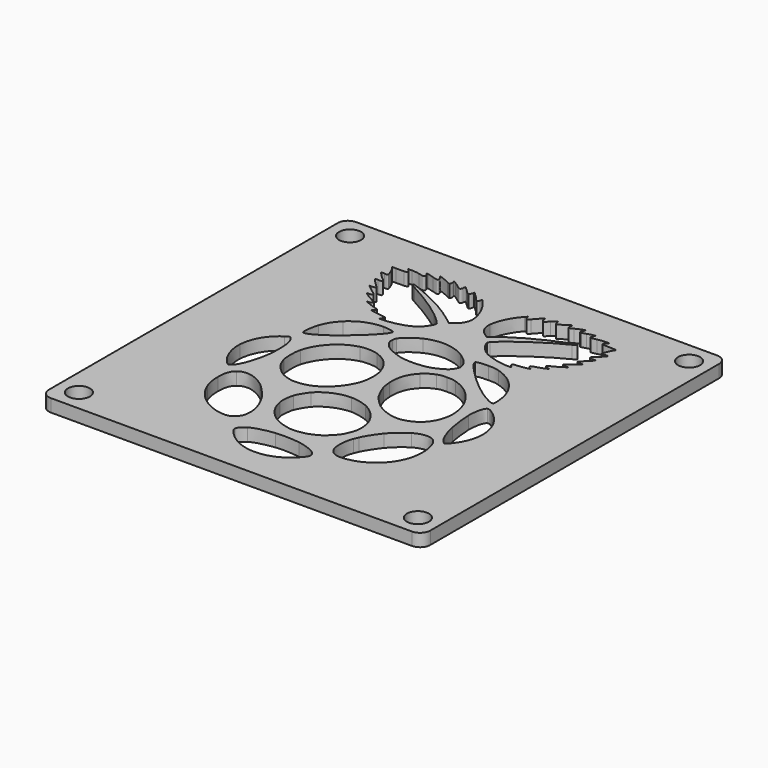
from build123d import *

# Parameters (mm, degrees)
F1_W     = 45
F1_H     = 45
F3_DEPTH = 1.5
F0_W     = 40
F0_H     = 40
F4_DEPTH = 1.5
F2_R     = 1.3
F5_DEPTH = 1.5
F6_R     = 1.2
F9_DEPTH = 28


# Not quite as in the source:
# - ends of sketch curves that miss each other by under 0.0002 mm in the source are joined
# - a feature names something its author has since deleted; it is built from what else it names


with BuildPart() as f3:
    # F1 (on Top) → F3 (new body)
    with BuildSketch(Plane.XY):
        Rectangle(F1_W, F1_H)
    extrude(amount=F3_DEPTH)

    # F0 (on Top) → F4 (join)
    with BuildSketch(Plane.XY):
        Rectangle(F0_W, F0_H)
    extrude(amount=F4_DEPTH)

    # F2 (on Top) → F5 (cut)
    with BuildSketch(Plane.XY):
        with Locations((-20, 20)):
            Circle(F2_R)
        with Locations((20, 20)):
            Circle(F2_R)
        with Locations((-20, -20)):
            Circle(F2_R)
        with Locations((20, -20)):
            Circle(F2_R)
    extrude(amount=F5_DEPTH, mode=Mode.SUBTRACT)

    # F6
    f6_edges = [f3.edges().sort_by_distance(p)[0] for p in [
        (22.5, 22.5, 0.75),
        (-22.5, 22.5, 0.75),
        (-22.5, -22.5, 0.75),
        (22.5, -22.5, 0.75),
    ]]
    fillet(f6_edges, radius=F6_R)

    # F8 (on offset) → F9 (cut)
    with BuildSketch(Plane.XY.offset(25)):
        with BuildLine():
            add(Edge.make_bspline(
                [(-0.887177, -19.067709), (-1.37051, -18.963367), (-1.920806, -18.777216), (-2.274089, -18.598552)],
                knots=[0, 0, 0, 0, 1, 1, 1, 1], degree=3))
            add(Edge.make_bspline(
                [(1.459681, -18.954491), (0.830557, -19.140329), (-0.298485, -19.194797), (-0.887177, -19.067709)],
                knots=[0, 0, 0, 0, 1, 1, 1, 1], degree=3))
            add(Edge.make_bspline(
                [(4.270525, -17.044889), (3.53259, -17.978447), (2.585341, -18.621978), (1.459681, -18.954491)],
                knots=[0, 0, 0, 0, 1, 1, 1, 1], degree=3))
            add(Edge.make_bspline(
                [(4.151263, -15.845306), (4.621657, -16.247946), (4.652807, -16.561266), (4.270525, -17.044889)],
                knots=[0, 0, 0, 0, 1, 1, 1, 1], degree=3))
            add(Edge.make_bspline(
                [(2.0744, -15.096764), (2.83072, -15.220852), (3.85158, -15.588789), (4.151263, -15.845306)],
                knots=[0, 0, 0, 0, 1, 1, 1, 1], degree=3))
            add(Edge.make_bspline(
                [(-0.779595, -15.005754), (-0.110166, -14.926798), (1.315549, -14.972262), (2.0744, -15.096764)],
                knots=[0, 0, 0, 0, 1, 1, 1, 1], degree=3))
            add(Edge.make_bspline(
                [(-3.491858, -15.740052), (-2.988685, -15.428195), (-1.929114, -15.141335), (-0.779595, -15.005754)],
                knots=[0, 0, 0, 0, 1, 1, 1, 1], degree=3))
            add(Edge.make_bspline(
                [(-4.28669, -16.671703), (-4.28669, -16.390931), (-4.000176, -16.055097), (-3.491858, -15.740052)],
                knots=[0, 0, 0, 0, 1, 1, 1, 1], degree=3))
            add(Edge.make_bspline(
                [(-2.274089, -18.598552), (-3.225122, -18.117593), (-4.28669, -17.101255), (-4.28669, -16.671703)],
                knots=[0, 0, 0, 0, 1, 1, 1, 1], degree=3))
        make_face()
        with BuildLine():
            add(Edge.make_bspline(
                [(-7.639187, -14.959263), (-9.375295, -14.593112), (-10.940378, -13.246308), (-11.591687, -11.558011)],
                knots=[0, 0, 0, 0, 1, 1, 1, 1], degree=3))
            add(Edge.make_bspline(
                [(-5.614103, -14.513096), (-6.04316, -15.058014), (-6.594745, -15.17954), (-7.639187, -14.959263)],
                knots=[0, 0, 0, 0, 1, 1, 1, 1], degree=3))
            add(Edge.make_bspline(
                [(-5.216704, -13.342755), (-5.262075, -13.965348), (-5.322169, -14.142328), (-5.614103, -14.513096)],
                knots=[0, 0, 0, 0, 1, 1, 1, 1], degree=3))
            add(Edge.make_bspline(
                [(-6.300441, -10.132584), (-5.552084, -11.291625), (-5.153311, -12.472844), (-5.216704, -13.342755)],
                knots=[0, 0, 0, 0, 1, 1, 1, 1], degree=3))
            add(Edge.make_bspline(
                [(-8.076125, -8.223123), (-7.617712, -8.559281), (-6.631616, -9.619669), (-6.300441, -10.132584)],
                knots=[0, 0, 0, 0, 1, 1, 1, 1], degree=3))
            add(Edge.make_bspline(
                [(-11.303389, -7.648184), (-10.556755, -7.048173), (-9.396515, -7.25487), (-8.076125, -8.223123)],
                knots=[0, 0, 0, 0, 1, 1, 1, 1], degree=3))
            add(Edge.make_bspline(
                [(-11.941857, -9.574962), (-11.939052, -8.581512), (-11.748239, -8.005675), (-11.303389, -7.648184)],
                knots=[0, 0, 0, 0, 1, 1, 1, 1], degree=3))
            add(Edge.make_bspline(
                [(-11.591687, -11.558011), (-11.837351, -10.921211), (-11.943954, -10.317508), (-11.941857, -9.574962)],
                knots=[0, 0, 0, 0, 1, 1, 1, 1], degree=3))
        make_face()
        with BuildLine():
            add(Edge.make_bspline(
                [(6.262145, -14.967016), (5.893137, -14.834758), (5.613918, -14.573111), (5.421003, -14.178806)],
                knots=[0, 0, 0, 0, 1, 1, 1, 1], degree=3))
            add(Edge.make_bspline(
                [(9.133644, -14.48583), (8.168538, -14.965389), (6.866406, -15.183591), (6.262145, -14.967016)],
                knots=[0, 0, 0, 0, 1, 1, 1, 1], degree=3))
            add(Edge.make_bspline(
                [(12.006219, -11.072921), (11.551716, -12.598138), (10.559015, -13.777568), (9.133644, -14.48583)],
                knots=[0, 0, 0, 0, 1, 1, 1, 1], degree=3))
            add(Edge.make_bspline(
                [(12.14776, -8.711004), (12.258855, -9.290003), (12.18871, -10.460516), (12.006219, -11.072921)],
                knots=[0, 0, 0, 0, 1, 1, 1, 1], degree=3))
            add(Edge.make_bspline(
                [(11.526211, -7.150542), (11.813997, -7.460815), (11.995142, -7.9156), (12.14776, -8.711004)],
                knots=[0, 0, 0, 0, 1, 1, 1, 1], degree=3))
            add(Edge.make_bspline(
                [(8.99643, -7.173879), (10.018251, -6.600622), (11.00768, -6.591495), (11.526211, -7.150542)],
                knots=[0, 0, 0, 0, 1, 1, 1, 1], degree=3))
            add(Edge.make_bspline(
                [(7.068817, -8.843622), (7.543457, -8.265319), (8.448742, -7.48114), (8.99643, -7.173879)],
                knots=[0, 0, 0, 0, 1, 1, 1, 1], degree=3))
            add(Edge.make_bspline(
                [(5.764471, -10.890116), (5.947246, -10.444129), (6.614661, -9.396967), (7.068817, -8.843622)],
                knots=[0, 0, 0, 0, 1, 1, 1, 1], degree=3))
            add(Edge.make_bspline(
                [(5.537969, -11.433611), (5.582241, -11.330639), (5.684167, -11.086066), (5.764471, -10.890116)],
                knots=[0, 0, 0, 0, 1, 1, 1, 1], degree=3))
            add(Edge.make_bspline(
                [(5.421003, -14.178806), (5.139993, -13.604443), (5.198884, -12.222282), (5.537969, -11.433611)],
                knots=[0, 0, 0, 0, 1, 1, 1, 1], degree=3))
        make_face()
        with BuildLine():
            add(Edge.make_bspline(
                [(-0.235604, -13.50576), (-1.520983, -13.321682), (-2.446325, -12.892636), (-3.164632, -12.147682)],
                knots=[0, 0, 0, 0, 1, 1, 1, 1], degree=3))
            add(Edge.make_bspline(
                [(1.294176, -13.368537), (0.827588, -13.48029), (0.064506, -13.548739), (-0.235604, -13.50576)],
                knots=[0, 0, 0, 0, 1, 1, 1, 1], degree=3))
            add(Edge.make_bspline(
                [(2.342359, -12.964243), (2.015156, -13.126896), (1.543474, -13.308828), (1.294176, -13.368537)],
                knots=[0, 0, 0, 0, 1, 1, 1, 1], degree=3))
            add(Edge.make_bspline(
                [(3.504831, -12.099096), (3.002423, -12.603148), (2.868984, -12.702458), (2.342359, -12.964243)],
                knots=[0, 0, 0, 0, 1, 1, 1, 1], degree=3))
            add(Edge.make_bspline(
                [(4.310692, -11.042532), (4.112024, -11.448654), (3.977986, -11.624393), (3.504831, -12.099096)],
                knots=[0, 0, 0, 0, 1, 1, 1, 1], degree=3))
            add(Edge.make_bspline(
                [(4.7003, -8.628597), (4.848256, -9.47946), (4.736451, -10.172181), (4.310692, -11.042532)],
                knots=[0, 0, 0, 0, 1, 1, 1, 1], degree=3))
            add(Edge.make_bspline(
                [(4.072547, -7.091122), (4.444928, -7.656361), (4.595264, -8.02456), (4.7003, -8.628597)],
                knots=[0, 0, 0, 0, 1, 1, 1, 1], degree=3))
            add(Edge.make_bspline(
                [(2.200713, -5.511063), (2.857354, -5.7868), (3.659134, -6.463601), (4.072547, -7.091122)],
                knots=[0, 0, 0, 0, 1, 1, 1, 1], degree=3))
            add(Edge.make_bspline(
                [(0.257769, -5.098998), (0.762084, -5.099054), (1.686404, -5.295094), (2.200713, -5.511063)],
                knots=[0, 0, 0, 0, 1, 1, 1, 1], degree=3))
            add(Edge.make_bspline(
                [(-3.303441, -6.648636), (-2.500624, -5.733191), (-1.042809, -5.098832), (0.257769, -5.098998)],
                knots=[0, 0, 0, 0, 1, 1, 1, 1], degree=3))
            add(Edge.make_bspline(
                [(-4.1749, -8.134608), (-4.037742, -7.735953), (-3.595159, -6.98128), (-3.303441, -6.648636)],
                knots=[0, 0, 0, 0, 1, 1, 1, 1], degree=3))
            add(Edge.make_bspline(
                [(-4.339107, -9.886584), (-4.409434, -9.514024), (-4.319552, -8.555046), (-4.1749, -8.134608)],
                knots=[0, 0, 0, 0, 1, 1, 1, 1], degree=3))
            add(Edge.make_bspline(
                [(-3.164632, -12.147682), (-3.832592, -11.454942), (-4.163202, -10.818452), (-4.339107, -9.886584)],
                knots=[0, 0, 0, 0, 1, 1, 1, 1], degree=3))
        make_face()
        with BuildLine():
            add(Edge.make_bspline(
                [(-13.180571, -6.694966), (-13.990038, -5.840955), (-14.48352, -4.449729), (-14.40991, -3.229206)],
                knots=[0, 0, 0, 0, 1, 1, 1, 1], degree=3))
            add(Edge.make_bspline(
                [(-12.795313, -7.025328), (-12.834983, -7.025328), (-13.008349, -6.876665), (-13.180571, -6.694966)],
                knots=[0, 0, 0, 0, 1, 1, 1, 1], degree=3))
            add(Edge.make_bspline(
                [(-11.056067, -2.860925), (-11.378643, -5.18677), (-12.146509, -7.025328), (-12.795313, -7.025328)],
                knots=[0, 0, 0, 0, 1, 1, 1, 1], degree=3))
            add(Edge.make_bspline(
                [(-11.089866, -0.450994), (-11.017705, -0.916083), (-10.996457, -2.431121), (-11.056067, -2.860925)],
                knots=[0, 0, 0, 0, 1, 1, 1, 1], degree=3))
            add(Edge.make_bspline(
                [(-11.767433, 0.793551), (-11.50836, 0.793551), (-11.193126, 0.214534), (-11.089866, -0.450994)],
                knots=[0, 0, 0, 0, 1, 1, 1, 1], degree=3))
            add(Edge.make_bspline(
                [(-12.195937, 0.576602), (-12.011923, 0.695924), (-11.819096, 0.793551), (-11.767433, 0.793551)],
                knots=[0, 0, 0, 0, 1, 1, 1, 1], degree=3))
            add(Edge.make_bspline(
                [(-14.40991, -3.229206), (-14.317171, -1.691471), (-13.483414, -0.258248), (-12.195937, 0.576602)],
                knots=[0, 0, 0, 0, 1, 1, 1, 1], degree=3))
        make_face()
        with BuildLine():
            add(Edge.make_bspline(
                [(12.400777, -6.735775), (11.971045, -6.358465), (11.479362, -5.183704), (11.231968, -3.943179)],
                knots=[0, 0, 0, 0, 1, 1, 1, 1], degree=3))
            add(Edge.make_bspline(
                [(12.643578, -6.912011), (12.620435, -6.912011), (12.511174, -6.832705), (12.400777, -6.735775)],
                knots=[0, 0, 0, 0, 1, 1, 1, 1], degree=3))
            add(Edge.make_bspline(
                [(13.724147, -5.604577), (13.393346, -6.220246), (12.821615, -6.912011), (12.643578, -6.912011)],
                knots=[0, 0, 0, 0, 1, 1, 1, 1], degree=3))
            add(Edge.make_bspline(
                [(12.291561, 0.591731), (14.29644, -0.911772), (14.882837, -3.448092), (13.724147, -5.604577)],
                knots=[0, 0, 0, 0, 1, 1, 1, 1], degree=3))
            add(Edge.make_bspline(
                [(11.424514, 0.968577), (11.585105, 1.041747), (11.838113, 0.931782), (12.291561, 0.591731)],
                knots=[0, 0, 0, 0, 1, 1, 1, 1], degree=3))
            add(Edge.make_bspline(
                [(10.897877, -1.140843), (10.89799, -0.089468), (11.128489, 0.833699), (11.424514, 0.968577)],
                knots=[0, 0, 0, 0, 1, 1, 1, 1], degree=3))
            add(Edge.make_bspline(
                [(11.231968, -3.943179), (11.042484, -2.99304), (10.897795, -1.779392), (10.897877, -1.140843)],
                knots=[0, 0, 0, 0, 1, 1, 1, 1], degree=3))
        make_face()
        with BuildLine():
            add(Edge.make_bspline(
                [(-6.666349, -5.76274), (-7.397165, -5.563072), (-7.812664, -5.318386), (-8.366105, -4.761759)],
                knots=[0, 0, 0, 0, 1, 1, 1, 1], degree=3))
            add(Edge.make_bspline(
                [(-5.589836, -5.868818), (-6.089609, -5.890241), (-6.261771, -5.873277), (-6.666349, -5.76274)],
                knots=[0, 0, 0, 0, 1, 1, 1, 1], degree=3))
            add(Edge.make_bspline(
                [(-3.037567, -4.927008), (-3.859885, -5.536619), (-4.651088, -5.828579), (-5.589836, -5.868818)],
                knots=[0, 0, 0, 0, 1, 1, 1, 1], degree=3))
            add(Edge.make_bspline(
                [(-1.048832, -2.213387), (-1.399312, -3.231715), (-2.170865, -4.284496), (-3.037567, -4.927008)],
                knots=[0, 0, 0, 0, 1, 1, 1, 1], degree=3))
            add(Edge.make_bspline(
                [(-0.96737, 0.699644), (-0.703326, -0.086928), (-0.737495, -1.308792), (-1.048832, -2.213387)],
                knots=[0, 0, 0, 0, 1, 1, 1, 1], degree=3))
            add(Edge.make_bspline(
                [(-3.42309, 3.239768), (-2.143037, 2.780187), (-1.411922, 2.023944), (-0.96737, 0.699644)],
                knots=[0, 0, 0, 0, 1, 1, 1, 1], degree=3))
            add(Edge.make_bspline(
                [(-5.480047, 3.292589), (-4.869522, 3.44673), (-3.932516, 3.422668), (-3.42309, 3.239768)],
                knots=[0, 0, 0, 0, 1, 1, 1, 1], degree=3))
            add(Edge.make_bspline(
                [(-9.344396, -0.617591), (-8.788871, 1.322296), (-7.294369, 2.834522), (-5.480047, 3.292589)],
                knots=[0, 0, 0, 0, 1, 1, 1, 1], degree=3))
            add(Edge.make_bspline(
                [(-9.366706, -3.05923), (-9.521893, -2.499388), (-9.509981, -1.195815), (-9.344396, -0.617591)],
                knots=[0, 0, 0, 0, 1, 1, 1, 1], degree=3))
            add(Edge.make_bspline(
                [(-8.366105, -4.761759), (-8.890736, -4.234108), (-9.175204, -3.750084), (-9.366706, -3.05923)],
                knots=[0, 0, 0, 0, 1, 1, 1, 1], degree=3))
        make_face()
        with BuildLine():
            add(Edge.make_bspline(
                [(5.685213, -5.683681), (4.999679, -5.613281), (4.164647, -5.284724), (3.47553, -4.814245)],
                knots=[0, 0, 0, 0, 1, 1, 1, 1], degree=3))
            add(Edge.make_bspline(
                [(6.77887, -5.631059), (6.39194, -5.717519), (6.135065, -5.729879), (5.685213, -5.683681)],
                knots=[0, 0, 0, 0, 1, 1, 1, 1], degree=3))
            add(Edge.make_bspline(
                [(9.388712, -0.341026), (10.142836, -2.830944), (9.00703, -5.133173), (6.77887, -5.631059)],
                knots=[0, 0, 0, 0, 1, 1, 1, 1], degree=3))
            add(Edge.make_bspline(
                [(5.739077, 3.408924), (7.469211, 2.86561), (8.84595, 1.451029), (9.388712, -0.341026)],
                knots=[0, 0, 0, 0, 1, 1, 1, 1], degree=3))
            add(Edge.make_bspline(
                [(4.608701, 3.538068), (5.19957, 3.540923), (5.386887, 3.519522), (5.739077, 3.408924)],
                knots=[0, 0, 0, 0, 1, 1, 1, 1], degree=3))
            add(Edge.make_bspline(
                [(3.509753, 3.381682), (3.857557, 3.517846), (3.978255, 3.535021), (4.608701, 3.538068)],
                knots=[0, 0, 0, 0, 1, 1, 1, 1], degree=3))
            add(Edge.make_bspline(
                [(2.221864, 2.567223), (2.575367, 2.931901), (2.92395, 3.152344), (3.509753, 3.381682)],
                knots=[0, 0, 0, 0, 1, 1, 1, 1], degree=3))
            add(Edge.make_bspline(
                [(1.115416, -0.566001), (1.045522, 0.71934), (1.397906, 1.717218), (2.221864, 2.567223)],
                knots=[0, 0, 0, 0, 1, 1, 1, 1], degree=3))
            add(Edge.make_bspline(
                [(1.256315, -1.614437), (1.198315, -1.396302), (1.13491, -0.924506), (1.115416, -0.566001)],
                knots=[0, 0, 0, 0, 1, 1, 1, 1], degree=3))
            add(Edge.make_bspline(
                [(2.15982, -3.512498), (1.91394, -3.182298), (1.368556, -2.036567), (1.256315, -1.614437)],
                knots=[0, 0, 0, 0, 1, 1, 1, 1], degree=3))
            add(Edge.make_bspline(
                [(3.47553, -4.814245), (3.1611, -4.599576), (2.432554, -3.878762), (2.15982, -3.512498)],
                knots=[0, 0, 0, 0, 1, 1, 1, 1], degree=3))
        make_face()
        with BuildLine():
            add(Edge.make_bspline(
                [(10.416201, 2.345395), (9.765312, 2.693907), (9.335171, 2.964027), (8.91475, 3.288278)],
                knots=[0, 0, 0, 0, 1, 1, 1, 1], degree=3))
            add(Edge.make_bspline(
                [(11.216192, 2.245104), (11.162124, 2.029681), (10.958074, 2.055262), (10.416201, 2.345395)],
                knots=[0, 0, 0, 0, 1, 1, 1, 1], degree=3))
            add(Edge.make_bspline(
                [(11.216588, 2.882513), (11.236851, 2.613562), (11.236667, 2.326728), (11.216192, 2.245104)],
                knots=[0, 0, 0, 0, 1, 1, 1, 1], degree=3))
            add(Edge.make_bspline(
                [(7.458432, 7.572423), (9.62561, 6.916458), (11.046244, 5.143608), (11.216588, 2.882513)],
                knots=[0, 0, 0, 0, 1, 1, 1, 1], degree=3))
            add(Edge.make_bspline(
                [(6.166811, 7.728751), (6.853439, 7.724014), (7.027005, 7.703009), (7.458432, 7.572423)],
                knots=[0, 0, 0, 0, 1, 1, 1, 1], degree=3))
            add(Edge.make_bspline(
                [(4.741901, 7.506008), (4.796308, 7.647789), (5.350255, 7.734383), (6.166811, 7.728751)],
                knots=[0, 0, 0, 0, 1, 1, 1, 1], degree=3))
            add(Edge.make_bspline(
                [(5.110777, 6.799356), (4.858896, 7.113128), (4.70458, 7.40875), (4.741901, 7.506008)],
                knots=[0, 0, 0, 0, 1, 1, 1, 1], degree=3))
            add(Edge.make_bspline(
                [(8.036543, 3.958679), (7.279806, 4.532045), (5.697985, 6.067863), (5.110777, 6.799356)],
                knots=[0, 0, 0, 0, 1, 1, 1, 1], degree=3))
            add(Edge.make_bspline(
                [(8.91475, 3.288278), (8.712196, 3.444499), (8.317003, 3.746179), (8.036543, 3.958679)],
                knots=[0, 0, 0, 0, 1, 1, 1, 1], degree=3))
        make_face()
        with BuildLine():
            add(Edge.make_bspline(
                [(-11.391275, 2.299636), (-11.494252, 2.56799), (-11.354362, 3.602861), (-11.123694, 4.279138)],
                knots=[0, 0, 0, 0, 1, 1, 1, 1], degree=3))
            add(Edge.make_bspline(
                [(-11.232042, 2.210014), (-11.300705, 2.210014), (-11.37236, 2.250344), (-11.391275, 2.299636)],
                knots=[0, 0, 0, 0, 1, 1, 1, 1], degree=3))
            add(Edge.make_bspline(
                [(-10.112701, 2.674987), (-10.455355, 2.455288), (-11.04581, 2.210014), (-11.232042, 2.210014)],
                knots=[0, 0, 0, 0, 1, 1, 1, 1], degree=3))
            add(Edge.make_bspline(
                [(-9.499276, 3.055627), (-9.670668, 2.952703), (-9.946709, 2.781416), (-10.112701, 2.674987)],
                knots=[0, 0, 0, 0, 1, 1, 1, 1], degree=3))
            add(Edge.make_bspline(
                [(-6.639739, 5.362827), (-7.53775, 4.527583), (-8.962803, 3.377787), (-9.499276, 3.055627)],
                knots=[0, 0, 0, 0, 1, 1, 1, 1], degree=3))
            add(Edge.make_bspline(
                [(-4.957272, 7.54926), (-4.778051, 7.370039), (-5.524177, 6.400419), (-6.639739, 5.362827)],
                knots=[0, 0, 0, 0, 1, 1, 1, 1], degree=3))
            add(Edge.make_bspline(
                [(-6.25059, 7.760561), (-5.723939, 7.758544), (-5.057705, 7.649693), (-4.957272, 7.54926)],
                knots=[0, 0, 0, 0, 1, 1, 1, 1], degree=3))
            add(Edge.make_bspline(
                [(-9.844138, 6.291024), (-8.887425, 7.240353), (-7.602654, 7.765745), (-6.25059, 7.760561)],
                knots=[0, 0, 0, 0, 1, 1, 1, 1], degree=3))
            add(Edge.make_bspline(
                [(-11.123694, 4.279138), (-10.854269, 5.069039), (-10.475596, 5.664438), (-9.844138, 6.291024)],
                knots=[0, 0, 0, 0, 1, 1, 1, 1], degree=3))
        make_face()
        with BuildLine():
            add(Edge.make_bspline(
                [(-0.75693, 3.913219), (-1.661555, 4.030979), (-2.894979, 4.537561), (-3.41168, 5.003555)],
                knots=[0, 0, 0, 0, 1, 1, 1, 1], degree=3))
            add(Edge.make_bspline(
                [(1.605798, 3.971855), (0.922233, 3.846833), (-0.059754, 3.822463), (-0.75693, 3.913219)],
                knots=[0, 0, 0, 0, 1, 1, 1, 1], degree=3))
            add(Edge.make_bspline(
                [(2.943425, 4.422067), (2.374586, 4.147585), (2.146049, 4.070665), (1.605798, 3.971855)],
                knots=[0, 0, 0, 0, 1, 1, 1, 1], degree=3))
            add(Edge.make_bspline(
                [(4.216517, 5.578006), (3.980659, 5.04481), (3.693325, 4.783917), (2.943425, 4.422067)],
                knots=[0, 0, 0, 0, 1, 1, 1, 1], degree=3))
            add(Edge.make_bspline(
                [(4.268538, 6.148803), (4.325273, 5.875514), (4.319344, 5.810464), (4.216517, 5.578006)],
                knots=[0, 0, 0, 0, 1, 1, 1, 1], degree=3))
            add(Edge.make_bspline(
                [(2.771734, 7.847433), (3.594347, 7.321914), (4.157729, 6.682567), (4.268538, 6.148803)],
                knots=[0, 0, 0, 0, 1, 1, 1, 1], degree=3))
            add(Edge.make_bspline(
                [(-1.943801, 8.212033), (-0.42835, 8.89197), (1.352178, 8.754301), (2.771734, 7.847433)],
                knots=[0, 0, 0, 0, 1, 1, 1, 1], degree=3))
            add(Edge.make_bspline(
                [(-3.858635, 6.692064), (-3.620796, 7.151995), (-2.729441, 7.85954), (-1.943801, 8.212033)],
                knots=[0, 0, 0, 0, 1, 1, 1, 1], degree=3))
            add(Edge.make_bspline(
                [(-3.987133, 6.204006), (-3.970143, 6.368625), (-3.912319, 6.588251), (-3.858635, 6.692064)],
                knots=[0, 0, 0, 0, 1, 1, 1, 1], degree=3))
            add(Edge.make_bspline(
                [(-3.8549, 5.580431), (-3.993254, 5.85546), (-4.013333, 5.950149), (-3.987133, 6.204006)],
                knots=[0, 0, 0, 0, 1, 1, 1, 1], degree=3))
            add(Edge.make_bspline(
                [(-3.41168, 5.003555), (-3.567636, 5.144205), (-3.764073, 5.399879), (-3.8549, 5.580431)],
                knots=[0, 0, 0, 0, 1, 1, 1, 1], degree=3))
        make_face()
        with BuildLine():
            add(Edge.make_bspline(
                [(-7.583908, 8.810406), (-7.605552, 8.833099), (-7.548185, 8.914838), (-7.456426, 8.992048)],
                knots=[0, 0, 0, 0, 1, 1, 1, 1], degree=3))
            add(Edge.make_bspline(
                [(-5.9005, 8.955461), (-6.468685, 8.832359), (-7.518565, 8.741893), (-7.583908, 8.810406)],
                knots=[0, 0, 0, 0, 1, 1, 1, 1], degree=3))
            add(Edge.make_bspline(
                [(-3.247876, 10.382302), (-3.752675, 9.672456), (-4.536049, 9.25108), (-5.9005, 8.955461)],
                knots=[0, 0, 0, 0, 1, 1, 1, 1], degree=3))
            add(Edge.make_bspline(
                [(-2.813568, 11.274492), (-2.813568, 11.104658), (-2.985819, 10.750807), (-3.247876, 10.382302)],
                knots=[0, 0, 0, 0, 1, 1, 1, 1], degree=3))
            add(Edge.make_bspline(
                [(-4.173373, 12.612296), (-3.530382, 12.090563), (-2.813568, 11.385346), (-2.813568, 11.274492)],
                knots=[0, 0, 0, 0, 1, 1, 1, 1], degree=3))
            add(Edge.make_bspline(
                [(-8.975184, 15.695384), (-7.157498, 14.731691), (-5.374354, 13.586791), (-4.173373, 12.612296)],
                knots=[0, 0, 0, 0, 1, 1, 1, 1], degree=3))
            add(Edge.make_bspline(
                [(-9.326446, 16.091357), (-9.566099, 16.091357), (-9.427627, 15.935259), (-8.975184, 15.695384)],
                knots=[0, 0, 0, 0, 1, 1, 1, 1], degree=3))
            add(Edge.make_bspline(
                [(-5.191011, 14.250973), (-6.397057, 14.923274), (-9.021798, 16.091357), (-9.326446, 16.091357)],
                knots=[0, 0, 0, 0, 1, 1, 1, 1], degree=3))
            add(Edge.make_bspline(
                [(-2.542429, 12.503854), (-3.10486, 12.95853), (-4.372307, 13.794593), (-5.191011, 14.250973)],
                knots=[0, 0, 0, 0, 1, 1, 1, 1], degree=3))
            Line((-2.542429, 12.503854), (-1.777539, 12.316211))
            add(Edge.make_bspline(
                [(-0.754494, 14.020254), (-0.756041, 13.332166), (-1.102995, 12.754256), (-1.777539, 12.316211)],
                knots=[0, 0, 0, 0, 1, 1, 1, 1], degree=3))
            add(Edge.make_bspline(
                [(-2.236226, 17.343044), (-1.406614, 16.440804), (-0.752353, 14.973619), (-0.754494, 14.020254)],
                knots=[0, 0, 0, 0, 1, 1, 1, 1], degree=3))
            Line((-2.236226, 17.343044), (-2.597227, 17.391871))
            add(Edge.make_bspline(
                [(-2.762855, 17.123708), (-2.718006, 17.132415), (-2.643474, 17.253089), (-2.597227, 17.391871)],
                knots=[0, 0, 0, 0, 1, 1, 1, 1], degree=3))
            add(Edge.make_bspline(
                [(-3.052306, 17.378671), (-2.937957, 17.229733), (-2.807704, 17.115), (-2.762855, 17.123708)],
                knots=[0, 0, 0, 0, 1, 1, 1, 1], degree=3))
            add(Edge.make_bspline(
                [(-4.023399, 18.314751), (-4.060666, 18.457259), (-3.36715, 17.788748), (-3.052306, 17.378671)],
                knots=[0, 0, 0, 0, 1, 1, 1, 1], degree=3))
            add(Edge.make_bspline(
                [(-4.22542, 17.764247), (-4.104771, 17.80254), (-3.979045, 18.14514), (-4.023399, 18.314751)],
                knots=[0, 0, 0, 0, 1, 1, 1, 1], degree=3))
            add(Edge.make_bspline(
                [(-4.781638, 18.186479), (-4.451461, 17.856302), (-4.299304, 17.740797), (-4.22542, 17.764247)],
                knots=[0, 0, 0, 0, 1, 1, 1, 1], degree=3))
            add(Edge.make_bspline(
                [(-5.299676, 18.640991), (-5.264736, 18.640991), (-5.031619, 18.436461), (-4.781638, 18.186479)],
                knots=[0, 0, 0, 0, 1, 1, 1, 1], degree=3))
            add(Edge.make_bspline(
                [(-5.363202, 18.425689), (-5.363202, 18.546968), (-5.33546, 18.640991), (-5.299676, 18.640991)],
                knots=[0, 0, 0, 0, 1, 1, 1, 1], degree=3))
            add(Edge.make_bspline(
                [(-5.572553, 18.074406), (-5.441507, 18.074406), (-5.363202, 18.205798), (-5.363202, 18.425689)],
                knots=[0, 0, 0, 0, 1, 1, 1, 1], degree=3))
            add(Edge.make_bspline(
                [(-5.986628, 18.348948), (-5.799241, 18.19795), (-5.612907, 18.074406), (-5.572553, 18.074406)],
                knots=[0, 0, 0, 0, 1, 1, 1, 1], degree=3))
            add(Edge.make_bspline(
                [(-6.61564, 18.780407), (-6.457071, 18.694103), (-6.174015, 18.499946), (-5.986628, 18.348948)],
                knots=[0, 0, 0, 0, 1, 1, 1, 1], degree=3))
            add(Edge.make_bspline(
                [(-6.83853, 18.815089), (-6.900272, 18.930456), (-6.887747, 18.928507), (-6.61564, 18.780407)],
                knots=[0, 0, 0, 0, 1, 1, 1, 1], degree=3))
            add(Edge.make_bspline(
                [(-6.902968, 18.255668), (-6.785133, 18.277983), (-6.74368, 18.63786), (-6.83853, 18.815089)],
                knots=[0, 0, 0, 0, 1, 1, 1, 1], degree=3))
            add(Edge.make_bspline(
                [(-7.240947, 18.391086), (-7.107293, 18.306714), (-6.955202, 18.245776), (-6.902968, 18.255668)],
                knots=[0, 0, 0, 0, 1, 1, 1, 1], degree=3))
            add(Edge.make_bspline(
                [(-8.429431, 18.867625), (-8.298125, 18.867625), (-7.46955, 18.535397), (-7.240947, 18.391086)],
                knots=[0, 0, 0, 0, 1, 1, 1, 1], degree=3))
            add(Edge.make_bspline(
                [(-8.342812, 18.693302), (-8.423488, 18.78918), (-8.462466, 18.867625), (-8.429431, 18.867625)],
                knots=[0, 0, 0, 0, 1, 1, 1, 1], degree=3))
            add(Edge.make_bspline(
                [(-8.289421, 18.187723), (-8.140904, 18.187723), (-8.17298, 18.491468), (-8.342812, 18.693302)],
                knots=[0, 0, 0, 0, 1, 1, 1, 1], degree=3))
            add(Edge.make_bspline(
                [(-8.898501, 18.350774), (-8.614818, 18.261096), (-8.340733, 18.187723), (-8.289421, 18.187723)],
                knots=[0, 0, 0, 0, 1, 1, 1, 1], degree=3))
            add(Edge.make_bspline(
                [(-9.640922, 18.554087), (-9.516273, 18.531943), (-9.182184, 18.440451), (-8.898501, 18.350774)],
                knots=[0, 0, 0, 0, 1, 1, 1, 1], degree=3))
            Line((-9.640922, 18.554087), (-9.740074, 18.458208))
            add(Edge.make_bspline(
                [(-9.612593, 18.141577), (-9.612593, 18.25064), (-9.663042, 18.375942), (-9.740074, 18.458208)],
                knots=[0, 0, 0, 0, 1, 1, 1, 1], degree=3))
            add(Edge.make_bspline(
                [(-10.320824, 18.074406), (-9.68754, 17.912439), (-9.612593, 17.919547), (-9.612593, 18.141577)],
                knots=[0, 0, 0, 0, 1, 1, 1, 1], degree=3))
            add(Edge.make_bspline(
                [(-11.240458, 18.187723), (-10.949351, 18.187723), (-10.591467, 18.143624), (-10.320824, 18.074406)],
                knots=[0, 0, 0, 0, 1, 1, 1, 1], degree=3))
            Line((-11.240458, 18.187723), (-11.514688, 17.996892))
            add(Edge.make_bspline(
                [(-11.723123, 17.592696), (-11.239516, 17.637563), (-11.204888, 17.704713), (-11.514688, 17.996892)],
                knots=[0, 0, 0, 0, 1, 1, 1, 1], degree=3))
            add(Edge.make_bspline(
                [(-12.621958, 17.573698), (-12.353525, 17.563188), (-11.949049, 17.571738), (-11.723123, 17.592696)],
                knots=[0, 0, 0, 0, 1, 1, 1, 1], degree=3))
            Line((-12.621958, 17.573698), (-12.971257, 17.411168))
            add(Edge.make_bspline(
                [(-12.446212, 16.212238), (-12.447118, 16.387367), (-12.793659, 17.178693), (-12.971257, 17.411168)],
                knots=[0, 0, 0, 0, 1, 1, 1, 1], degree=3))
            add(Edge.make_bspline(
                [(-12.8138, 16.117595), (-12.453047, 16.078962), (-12.445534, 16.080896), (-12.446212, 16.212238)],
                knots=[0, 0, 0, 0, 1, 1, 1, 1], degree=3))
            add(Edge.make_bspline(
                [(-13.182081, 16.09166), (-13.182081, 16.138394), (-13.077069, 16.145789), (-12.8138, 16.117595)],
                knots=[0, 0, 0, 0, 1, 1, 1, 1], degree=3))
            add(Edge.make_bspline(
                [(-12.336475, 15.213148), (-12.624692, 15.424566), (-13.182081, 16.003644), (-13.182081, 16.09166)],
                knots=[0, 0, 0, 0, 1, 1, 1, 1], degree=3))
            add(Edge.make_bspline(
                [(-12.119325, 14.901526), (-12.108141, 15.010242), (-12.158624, 15.082688), (-12.336475, 15.213148)],
                knots=[0, 0, 0, 0, 1, 1, 1, 1], degree=3))
            add(Edge.make_bspline(
                [(-12.510271, 14.759879), (-12.150465, 14.759879), (-12.133256, 14.766114), (-12.119325, 14.901526)],
                knots=[0, 0, 0, 0, 1, 1, 1, 1], degree=3))
            Line((-12.510271, 14.759879), (-12.776285, 14.605113))
            add(Edge.make_bspline(
                [(-12.187888, 14.010198), (-12.450809, 14.25228), (-12.715587, 14.519992), (-12.776285, 14.605113)],
                knots=[0, 0, 0, 0, 1, 1, 1, 1], degree=3))
            add(Edge.make_bspline(
                [(-11.709405, 13.505289), (-11.709631, 13.540907), (-11.924968, 13.768117), (-12.187888, 14.010198)],
                knots=[0, 0, 0, 0, 1, 1, 1, 1], degree=3))
            add(Edge.make_bspline(
                [(-12.152697, 13.369329), (-11.845722, 13.372134), (-11.708777, 13.414135), (-11.709405, 13.505289)],
                knots=[0, 0, 0, 0, 1, 1, 1, 1], degree=3))
            Line((-12.152697, 13.369329), (-12.162227, 13.140631))
            add(Edge.make_bspline(
                [(-11.470076, 12.618957), (-11.710529, 12.78142), (-12.021997, 13.016174), (-12.162227, 13.140631)],
                knots=[0, 0, 0, 0, 1, 1, 1, 1], degree=3))
            add(Edge.make_bspline(
                [(-11.444465, 12.066565), (-10.888261, 12.071364), (-10.895655, 12.230844), (-11.470076, 12.618957)],
                knots=[0, 0, 0, 0, 1, 1, 1, 1], degree=3))
            Line((-11.444465, 12.066565), (-11.510654, 11.923649))
            add(Edge.make_bspline(
                [(-10.240111, 11.17892), (-10.52654, 11.291433), (-11.28244, 11.734503), (-11.510654, 11.923649)],
                knots=[0, 0, 0, 0, 1, 1, 1, 1], degree=3))
            add(Edge.make_bspline(
                [(-10.480324, 10.76295), (-9.991013, 10.769741), (-9.844469, 11.023507), (-10.240111, 11.17892)],
                knots=[0, 0, 0, 0, 1, 1, 1, 1], degree=3))
            Line((-10.480324, 10.76295), (-10.462471, 10.655618))
            add(Edge.make_bspline(
                [(-8.989349, 10.145724), (-9.54331, 10.307189), (-10.296553, 10.567911), (-10.462471, 10.655618)],
                knots=[0, 0, 0, 0, 1, 1, 1, 1], degree=3))
            add(Edge.make_bspline(
                [(-9.074337, 9.776533), (-8.808668, 9.906316), (-8.768382, 10.081318), (-8.989349, 10.145724)],
                knots=[0, 0, 0, 0, 1, 1, 1, 1], degree=3))
            Line((-9.074337, 9.776533), (-9.046007, 9.590982))
            add(Edge.make_bspline(
                [(-8.224458, 9.456601), (-8.53608, 9.489351), (-8.905777, 9.549822), (-9.046007, 9.590982)],
                knots=[0, 0, 0, 0, 1, 1, 1, 1], degree=3))
            add(Edge.make_bspline(
                [(-7.289593, 9.238142), (-7.289593, 9.355611), (-7.310923, 9.360596), (-8.224458, 9.456601)],
                knots=[0, 0, 0, 0, 1, 1, 1, 1], degree=3))
            add(Edge.make_bspline(
                [(-7.456426, 8.992048), (-7.364668, 9.069258), (-7.289593, 9.18), (-7.289593, 9.238142)],
                knots=[0, 0, 0, 0, 1, 1, 1, 1], degree=3))
        make_face()
        Polygon((-9.300971, 9.66582), (-9.046007, 9.590982), (-9.074337, 9.776533), align=None)
        Polygon((-10.660776, 10.760446), (-10.462471, 10.655618), (-10.480324, 10.76295), align=None)
        Polygon((-1.777539, 12.316211), (-2.542429, 12.503854), (-2.072986, 12.124349), align=None)
        Polygon((-11.680629, 12.064525), (-11.510654, 11.923649), (-11.444465, 12.066565), align=None)
        Polygon((-2.597227, 17.391871), (-2.236226, 17.343044), (-2.513143, 17.644203), align=None)
        Polygon((-12.41719, 13.366915), (-12.162227, 13.140631), (-12.152697, 13.369329), align=None)
        Polygon((-12.886644, 14.759879), (-12.776285, 14.605113), (-12.510271, 14.759879), align=None)
        Polygon((-13.11002, 17.592808), (-12.971257, 17.411168), (-12.621958, 17.573698), align=None)
        Polygon((-11.717027, 18.187723), (-11.514688, 17.996892), (-11.240458, 18.187723), align=None)
        Polygon((-9.740074, 18.458208), (-9.640922, 18.554087), (-9.867556, 18.59435), align=None)
        with BuildLine():
            add(Edge.make_bspline(
                [(6.678906, 8.872284), (6.000035, 8.977778), (5.237201, 9.200614), (4.738118, 9.439219)],
                knots=[0, 0, 0, 0, 1, 1, 1, 1], degree=3))
            add(Edge.make_bspline(
                [(7.970238, 8.819974), (7.90965, 8.759386), (7.227638, 8.787013), (6.678906, 8.872284)],
                knots=[0, 0, 0, 0, 1, 1, 1, 1], degree=3))
            add(Edge.make_bspline(
                [(7.838034, 8.960788), (7.931409, 8.904003), (7.9909, 8.840637), (7.970238, 8.819974)],
                knots=[0, 0, 0, 0, 1, 1, 1, 1], degree=3))
            add(Edge.make_bspline(
                [(7.668262, 9.200449), (7.668262, 9.109654), (7.725039, 9.029504), (7.838034, 8.960788)],
                knots=[0, 0, 0, 0, 1, 1, 1, 1], degree=3))
            add(Edge.make_bspline(
                [(8.118743, 9.405649), (7.759491, 9.405649), (7.668262, 9.364093), (7.668262, 9.200449)],
                knots=[0, 0, 0, 0, 1, 1, 1, 1], degree=3))
            add(Edge.make_bspline(
                [(9.485626, 9.622779), (9.266533, 9.541734), (8.409858, 9.405649), (8.118743, 9.405649)],
                knots=[0, 0, 0, 0, 1, 1, 1, 1], degree=3))
            add(Edge.make_bspline(
                [(9.408492, 9.771961), (9.61316, 9.67484), (9.615279, 9.670741), (9.485626, 9.622779)],
                knots=[0, 0, 0, 0, 1, 1, 1, 1], degree=3))
            add(Edge.make_bspline(
                [(9.198256, 9.992852), (9.198086, 9.908799), (9.262336, 9.841317), (9.408492, 9.771961)],
                knots=[0, 0, 0, 0, 1, 1, 1, 1], degree=3))
            add(Edge.make_bspline(
                [(9.762379, 10.275586), (9.274939, 10.135806), (9.198441, 10.097466), (9.198256, 9.992852)],
                knots=[0, 0, 0, 0, 1, 1, 1, 1], degree=3))
            add(Edge.make_bspline(
                [(10.654537, 10.597029), (10.474, 10.509175), (10.072529, 10.364526), (9.762379, 10.275586)],
                knots=[0, 0, 0, 0, 1, 1, 1, 1], degree=3))
            add(Edge.make_bspline(
                [(10.801312, 10.761107), (10.973217, 10.756994), (10.965477, 10.74834), (10.654537, 10.597029)],
                knots=[0, 0, 0, 0, 1, 1, 1, 1], degree=3))
            add(Edge.make_bspline(
                [(10.334959, 10.987015), (10.330369, 10.876702), (10.556922, 10.766957), (10.801312, 10.761107)],
                knots=[0, 0, 0, 0, 1, 1, 1, 1], degree=3))
            add(Edge.make_bspline(
                [(10.88738, 11.345907), (10.545988, 11.178636), (10.337289, 11.04305), (10.334959, 10.987015)],
                knots=[0, 0, 0, 0, 1, 1, 1, 1], degree=3))
            add(Edge.make_bspline(
                [(11.746943, 11.841669), (11.575955, 11.716859), (11.189151, 11.493766), (10.88738, 11.345907)],
                knots=[0, 0, 0, 0, 1, 1, 1, 1], degree=3))
            Line((11.746943, 11.841669), (11.831931, 12.069374))
            add(Edge.make_bspline(
                [(11.351067, 12.215128), (11.351067, 12.123148), (11.525009, 12.070425), (11.831931, 12.069374)],
                knots=[0, 0, 0, 0, 1, 1, 1, 1], degree=3))
            add(Edge.make_bspline(
                [(11.76197, 12.569056), (11.535974, 12.416555), (11.351067, 12.257287), (11.351067, 12.215128)],
                knots=[0, 0, 0, 0, 1, 1, 1, 1], degree=3))
            add(Edge.make_bspline(
                [(12.456038, 13.106789), (12.300298, 12.963537), (11.987968, 12.721557), (11.76197, 12.569056)],
                knots=[0, 0, 0, 0, 1, 1, 1, 1], degree=3))
            Line((12.456038, 13.106789), (12.474708, 13.369497))
            add(Edge.make_bspline(
                [(12.03097, 13.487676), (12.03097, 13.413602), (12.187399, 13.371941), (12.474708, 13.369497)],
                knots=[0, 0, 0, 0, 1, 1, 1, 1], degree=3))
            add(Edge.make_bspline(
                [(12.625885, 14.113631), (12.298681, 13.795286), (12.03097, 13.513607), (12.03097, 13.487676)],
                knots=[0, 0, 0, 0, 1, 1, 1, 1], degree=3))
            add(Edge.make_bspline(
                [(13.220902, 14.72616), (13.220846, 14.707613), (12.953088, 14.431975), (12.625885, 14.113631)],
                knots=[0, 0, 0, 0, 1, 1, 1, 1], degree=3))
            add(Edge.make_bspline(
                [(12.895116, 14.744082), (13.074355, 14.752772), (13.220959, 14.744706), (13.220902, 14.72616)],
                knots=[0, 0, 0, 0, 1, 1, 1, 1], degree=3))
            add(Edge.make_bspline(
                [(12.818875, 15.322204), (12.285665, 14.894531), (12.309251, 14.715681), (12.895116, 14.744082)],
                knots=[0, 0, 0, 0, 1, 1, 1, 1], degree=3))
            add(Edge.make_bspline(
                [(13.527687, 16.081196), (13.396392, 15.861415), (13.113571, 15.558572), (12.818875, 15.322204)],
                knots=[0, 0, 0, 0, 1, 1, 1, 1], degree=3))
            add(Edge.make_bspline(
                [(13.169959, 16.116369), (13.495791, 16.148476), (13.563879, 16.141781), (13.527687, 16.081196)],
                knots=[0, 0, 0, 0, 1, 1, 1, 1], degree=3))
            add(Edge.make_bspline(
                [(12.767531, 16.172963), (12.767531, 16.087717), (12.813531, 16.081248), (13.169959, 16.116369)],
                knots=[0, 0, 0, 0, 1, 1, 1, 1], degree=3))
            add(Edge.make_bspline(
                [(13.254292, 17.311733), (13.093955, 17.075464), (12.767531, 16.311799), (12.767531, 16.172963)],
                knots=[0, 0, 0, 0, 1, 1, 1, 1], degree=3))
            add(Edge.make_bspline(
                [(13.390775, 17.538666), (13.390775, 17.524468), (13.329358, 17.422349), (13.254292, 17.311733)],
                knots=[0, 0, 0, 0, 1, 1, 1, 1], degree=3))
            add(Edge.make_bspline(
                [(12.810025, 17.564971), (13.129437, 17.564688), (13.390775, 17.552863), (13.390775, 17.538666)],
                knots=[0, 0, 0, 0, 1, 1, 1, 1], degree=3))
            add(Edge.make_bspline(
                [(11.63436, 17.697464), (11.63436, 17.617409), (12.094276, 17.565578), (12.810025, 17.564971)],
                knots=[0, 0, 0, 0, 1, 1, 1, 1], degree=3))
            add(Edge.make_bspline(
                [(11.844164, 17.972864), (11.728772, 17.854692), (11.63436, 17.730762), (11.63436, 17.697464)],
                knots=[0, 0, 0, 0, 1, 1, 1, 1], degree=3))
            Line((11.844164, 17.972864), (11.598264, 18.187723))
            add(Edge.make_bspline(
                [(10.699494, 18.074406), (10.962242, 18.141606), (11.32802, 18.187723), (11.598264, 18.187723)],
                knots=[0, 0, 0, 0, 1, 1, 1, 1], degree=3))
            add(Edge.make_bspline(
                [(10.095516, 17.961089), (10.184018, 17.961089), (10.455808, 18.012081), (10.699494, 18.074406)],
                knots=[0, 0, 0, 0, 1, 1, 1, 1], degree=3))
            add(Edge.make_bspline(
                [(9.934604, 18.133639), (9.934604, 17.981848), (9.953964, 17.961089), (10.095516, 17.961089)],
                knots=[0, 0, 0, 0, 1, 1, 1, 1], degree=3))
            add(Edge.make_bspline(
                [(10.079144, 18.450731), (9.987478, 18.359064), (9.934604, 18.24307), (9.934604, 18.133639)],
                knots=[0, 0, 0, 0, 1, 1, 1, 1], degree=3))
            Line((10.079144, 18.450731), (9.979991, 18.555363))
            add(Edge.make_bspline(
                [(9.207376, 18.347381), (9.498284, 18.439822), (9.84596, 18.533414), (9.979991, 18.555363)],
                knots=[0, 0, 0, 0, 1, 1, 1, 1], degree=3))
            add(Edge.make_bspline(
                [(8.598297, 18.210066), (8.642383, 18.193148), (8.916469, 18.25494), (9.207376, 18.347381)],
                knots=[0, 0, 0, 0, 1, 1, 1, 1], degree=3))
            add(Edge.make_bspline(
                [(8.658612, 18.662198), (8.501334, 18.430437), (8.47809, 18.256193), (8.598297, 18.210066)],
                knots=[0, 0, 0, 0, 1, 1, 1, 1], degree=3))
            Line((8.658612, 18.662198), (8.644447, 18.831446))
            add(Edge.make_bspline(
                [(7.680995, 18.440385), (8.029875, 18.632153), (8.334403, 18.75576), (8.644447, 18.831446)],
                knots=[0, 0, 0, 0, 1, 1, 1, 1], degree=3))
            add(Edge.make_bspline(
                [(7.247435, 18.244381), (7.289771, 18.244381), (7.484873, 18.332583), (7.680995, 18.440385)],
                knots=[0, 0, 0, 0, 1, 1, 1, 1], degree=3))
            add(Edge.make_bspline(
                [(7.192682, 18.802363), (7.051144, 18.60029), (7.086068, 18.244381), (7.247435, 18.244381)],
                knots=[0, 0, 0, 0, 1, 1, 1, 1], degree=3))
            Line((7.192682, 18.802363), (7.000695, 18.788889))
            add(Edge.make_bspline(
                [(6.34516, 18.359946), (6.55006, 18.516993), (6.845051, 18.710018), (7.000695, 18.788889)],
                knots=[0, 0, 0, 0, 1, 1, 1, 1], degree=3))
            add(Edge.make_bspline(
                [(5.88417, 18.074406), (5.932815, 18.074406), (6.14026, 18.202899), (6.34516, 18.359946)],
                knots=[0, 0, 0, 0, 1, 1, 1, 1], degree=3))
            add(Edge.make_bspline(
                [(5.685213, 18.503033), (5.685213, 18.291149), (5.78582, 18.074406), (5.88417, 18.074406)],
                knots=[0, 0, 0, 0, 1, 1, 1, 1], degree=3))
            add(Edge.make_bspline(
                [(5.628142, 18.640991), (5.659531, 18.640991), (5.685213, 18.57891), (5.685213, 18.503033)],
                knots=[0, 0, 0, 0, 1, 1, 1, 1], degree=3))
            add(Edge.make_bspline(
                [(5.122046, 18.187723), (5.369009, 18.43702), (5.596752, 18.640991), (5.628142, 18.640991)],
                knots=[0, 0, 0, 0, 1, 1, 1, 1], degree=3))
            add(Edge.make_bspline(
                [(4.631158, 17.734454), (4.654183, 17.734454), (4.875082, 17.938425), (5.122046, 18.187723)],
                knots=[0, 0, 0, 0, 1, 1, 1, 1], degree=3))
            add(Edge.make_bspline(
                [(4.382067, 18.139846), (4.382067, 17.939941), (4.508328, 17.734454), (4.631158, 17.734454)],
                knots=[0, 0, 0, 0, 1, 1, 1, 1], degree=3))
            add(Edge.make_bspline(
                [(4.334389, 18.357698), (4.360612, 18.357698), (4.382067, 18.259664), (4.382067, 18.139846)],
                knots=[0, 0, 0, 0, 1, 1, 1, 1], degree=3))
            add(Edge.make_bspline(
                [(3.4191, 17.406227), (3.689429, 17.746762), (4.277133, 18.357698), (4.334389, 18.357698)],
                knots=[0, 0, 0, 0, 1, 1, 1, 1], degree=3))
            add(Edge.make_bspline(
                [(2.932791, 17.422832), (3.023993, 17.101503), (3.173156, 17.09641), (3.4191, 17.406227)],
                knots=[0, 0, 0, 0, 1, 1, 1, 1], degree=3))
            Line((2.932791, 17.422832), (2.655044, 17.422832))
            add(Edge.make_bspline(
                [(1.112054, 14.214829), (1.182671, 15.186875), (1.843752, 16.561318), (2.655044, 17.422832)],
                knots=[0, 0, 0, 0, 1, 1, 1, 1], degree=3))
            add(Edge.make_bspline(
                [(2.051953, 12.365434), (1.363103, 12.828402), (1.055328, 13.433994), (1.112054, 14.214829)],
                knots=[0, 0, 0, 0, 1, 1, 1, 1], degree=3))
            Line((2.051953, 12.365434), (2.617561, 12.295646))
            add(Edge.make_bspline(
                [(9.226372, 15.954559), (6.767785, 15.025725), (4.173107, 13.589203), (2.617561, 12.295646)],
                knots=[0, 0, 0, 0, 1, 1, 1, 1], degree=3))
            add(Edge.make_bspline(
                [(9.835451, 16.147611), (9.780918, 16.147384), (9.506832, 16.060515), (9.226372, 15.954559)],
                knots=[0, 0, 0, 0, 1, 1, 1, 1], degree=3))
            add(Edge.make_bspline(
                [(9.552159, 15.813855), (9.916879, 15.993625), (10.04832, 16.148479), (9.835451, 16.147611)],
                knots=[0, 0, 0, 0, 1, 1, 1, 1], degree=3))
            add(Edge.make_bspline(
                [(3.314021, 11.494661), (4.28061, 12.610062), (7.315681, 14.7115), (9.552159, 15.813855)],
                knots=[0, 0, 0, 0, 1, 1, 1, 1], degree=3))
            Line((3.314021, 11.494661), (3.222308, 11.043812))
            add(Edge.make_bspline(
                [(4.738118, 9.439219), (4.063567, 9.761714), (3.442818, 10.41882), (3.222308, 11.043812)],
                knots=[0, 0, 0, 0, 1, 1, 1, 1], degree=3))
        make_face()
        Polygon((3.1358, 11.289002), (3.222308, 11.043812), (3.314021, 11.494661), align=None)
        Polygon((2.411165, 12.124012), (2.617561, 12.295646), (2.051953, 12.365434), align=None)
        Polygon((2.868466, 17.649467), (2.655044, 17.422832), (2.932791, 17.422832), align=None)
        Polygon((11.831931, 12.069374), (11.746943, 11.841669), (12.057831, 12.068598), align=None)
        Polygon((12.474708, 13.369497), (12.456038, 13.106789), (12.739202, 13.367248), align=None)
        Polygon((7.283686, 18.932291), (7.000695, 18.788889), (7.192682, 18.802363), align=None)
        Polygon((8.799083, 18.869194), (8.644447, 18.831446), (8.658612, 18.662198), align=None)
        Polygon((10.223684, 18.59527), (9.979991, 18.555363), (10.079144, 18.450731), align=None)
        Polygon((11.598264, 18.187723), (11.844164, 17.972864), (12.053968, 18.187723), align=None)
    extrude(amount=-F9_DEPTH, mode=Mode.SUBTRACT)


solid = f3.part
